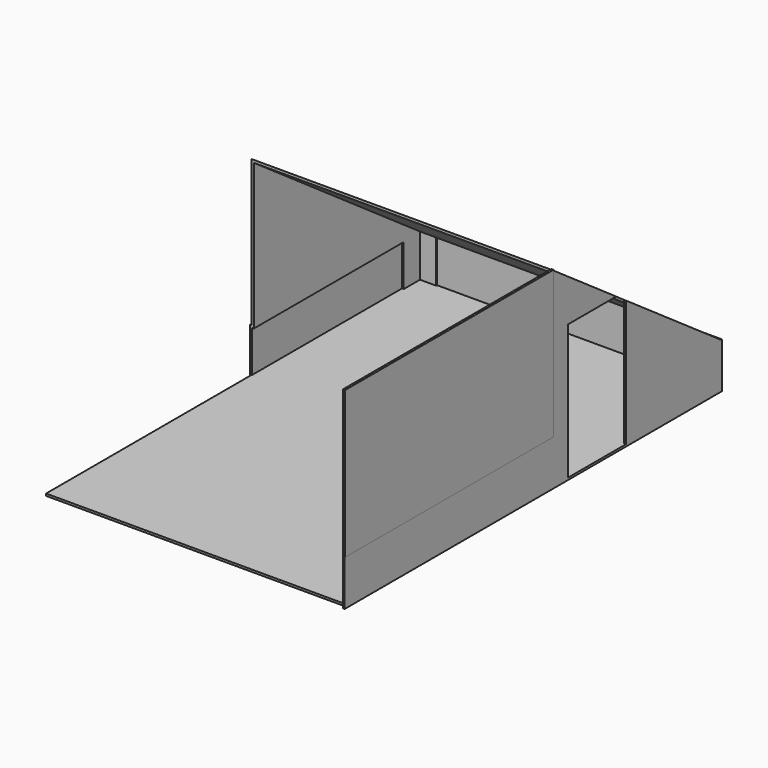
from build123d import *

# Parameters (mm, degrees)
F1_DEPTH    = 535
F3_DEPTH    = 3530
F4_T        = 25
F4_T3_DEPTH = 585
F4_T5_DEPTH = 3390
F4_T7_DEPTH = 2270
F5_W        = 3050
F5_H        = 1722.6878070831
F6_DEPTH    = 25
F7_W        = 850
F7_H        = 1580
F8_DEPTH    = 25
F9_W        = 3505
F9_H        = 3008.0275535583
F10_DEPTH   = 25


# Not quite as in the source:
# - a shell that OpenCascade refuses in one call is made with other operations: the cavity is built on its own and cut out


with BuildPart() as f1:
    # F0 (on Top) → F1 (new body)
    with BuildSketch(Plane.XY):
        Polygon((-20, 0), (0, 0), (0, 2200), (210, 2200), (210, 2450), (3510, 2450), (3510, -3050), (3530, -3050), (3530, 2470), (190, 2470), (190, 2220), (-20, 2220), align=None)
    extrude(amount=F1_DEPTH)

    # F2 (on face) → F3 (join)
    with BuildSketch(Plane.YZ):
        Polygon((0, 2249.3429109028), (0, 0), (2457.4198722839, 0), (2457.4198722839, 535), align=None)
    extrude(amount=F3_DEPTH)

    # F4: shell of thickness 25, made by hand


with BuildPart() as f4_core1:
    # F4_t2: copy of F1
    add(f1.part)

    # the walls: a layer under each face that stays
    f4_faces = [f4_core1.faces().sort_by_distance(p)[0] for p in [
        (571.6666666667, 1550, 0),
        (-10, 2220, 267.5),
        (95, 2457.4198722839, 267.5),
        (190, 2463.709936142, 267.5),
        (1860, 2463.709936142, 535),
        (1860, 2470, 267.5),
        (3520, -3050, 267.5),
        (3510, -1525, 267.5),
        (3520, -1525, 535),
        (3530, -2130, 374.8904851505),
        (1765, 1228.709936142, 1392.1714554514),
        (0, 1228.709936142, 1124.6714554514),
        (-10, 1110, 535),
        (-20, 1110, 267.5),
    ]]
    thicken(f4_faces, amount=-F4_T, mode=Mode.SUBTRACT)

    # F4_s4 → F4_t3 (cut)
    with BuildSketch(Plane.XY.offset(-25)):
        Polygon((-0.25, 2220.25), (0, 2195), (25, 2195), (25, 2220), align=None)
        Polygon((189.75, 2457.6698722839), (190, 2432.4198722839), (215, 2432.4198722839), (215, 2457.4198722839), align=None)
    extrude(amount=F4_T3_DEPTH, mode=Mode.SUBTRACT)

    # F4_s6 → F4_t5 (cut)
    with BuildSketch(Plane.YZ.offset(165)):
        Polygon((2457.5629100467, 535.455037066), (2457.4198722839, 510), (2449.5612947416, 510), (2443.1160960124, 514.4962933992), align=None)
    extrude(amount=F4_T5_DEPTH, mode=Mode.SUBTRACT)

    # F4_s8 → F4_t7 (cut)
    with BuildSketch(Plane.XZ.offset(-2245)):
        Polygon((-0.25, 535.25), (25, 535), (25, 510), (0, 510), align=None)
    extrude(amount=F4_T7_DEPTH, mode=Mode.SUBTRACT)


with BuildPart() as f1_1:
    add(f1.part)

    # what is left inside the walls is the cavity
    f4_cavity = [f4_core1.part.solids().sort_by_distance(p)[0] for p in [
        (2345, 1221.41501, 1366.473418),
    ]]
    add(f4_cavity, mode=Mode.SUBTRACT)

    # F5 (on face) → F6 (join)
    with BuildSketch(Plane(origin=(3510, 0, 0), x_dir=(0, -1, 0), z_dir=(-1, 0, 0))):
        with Locations((1525, 1396.3439035416)):
            Rectangle(F5_W, F5_H)
    extrude(amount=-F6_DEPTH)

    # F7 (on face) → F8 (cut)
    with BuildSketch(Plane(origin=(3505, 0, 0), x_dir=(0, -1, 0), z_dir=(-1, 0, 0))):
        with Locations((-640, 815)):
            Rectangle(F7_W, F7_H)
    extrude(amount=-F8_DEPTH, mode=Mode.SUBTRACT)

    # F9 (on face) → F10 (join)
    with BuildSketch(Plane.XY.offset(25)):
        with Locations((1752.5, -1504.0137767792)):
            Rectangle(F9_W, F9_H)
    extrude(amount=-F10_DEPTH)


solid = f1_1.part
